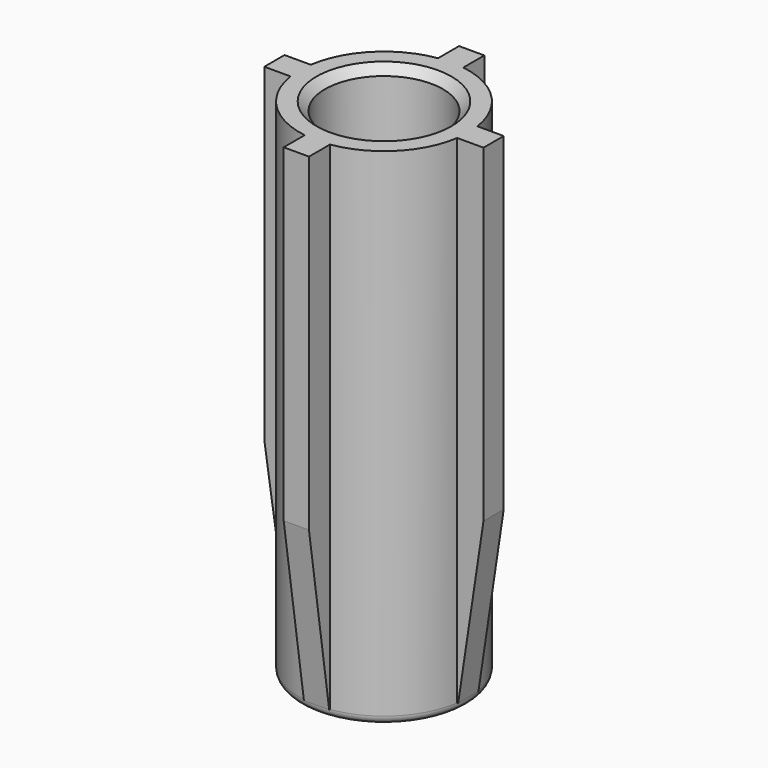
from build123d import *

# Parameters (mm, degrees)
F1_R        = 5
F1_R_2      = 3.5
F2_DEPTH    = 30
F4_W        = 1.5
F4_H        = 2.639524132
F5_DEPTH    = 29.5
F6_COUNT    = 4
F8_R        = 3.5
F8_R_2      = 1.75
F9_DEPTH    = 1.5
F10_SIZE2   = 1.49999
F10_SIZE    = 9.99999
F10_2_SIZE2 = 1.49999
F10_2_SIZE  = 9.99999
F10_3_SIZE2 = 1.49999
F10_3_SIZE  = 9.99999
F10_4_SIZE2 = 1.49999
F10_4_SIZE  = 9.99999
F11_SIZE    = 0.5
F12_R       = 0.49999


# Not quite as in the source:
# - a fillet or chamfer is up to 0.001 mm smaller than in the source, because OpenCascade refuses the exact size


with BuildPart() as f2:
    # F1 (on offset) → F2 (new body)
    with BuildSketch(Plane.XY):
        with Locations((-25, 25)):
            Circle(F1_R)
        with Locations((-25, 25)):
            Circle(F1_R_2, mode=Mode.SUBTRACT)
    extrude(amount=-F2_DEPTH)

    # F4 (on offset) → F5 (join)
    with BuildSketch(Plane.XY):
        with Locations((-25, 30.180237934)):
            Rectangle(F4_W, F4_H)
    extrude(amount=-F5_DEPTH)

    # F6: F2 ×4 about axis
    f6_axis = Axis((-25, 25, 0), (0, 0, 1))


with BuildPart() as f2_1:
    add(f2.part)
    for i in range(1, F6_COUNT):
        add(f2.part.rotate(f6_axis, i * 360 / F6_COUNT))

    # F8 (on offset) → F9 (join)
    with BuildSketch(Plane.XY.offset(-30)):
        with Locations((-25, 25)):
            Circle(F8_R)
        with Locations((-25, 25)):
            Circle(F8_R_2, mode=Mode.SUBTRACT)
    extrude(amount=F9_DEPTH)

    # F10 (size 10 and 1.5 in the source; OpenCascade refuses exactly that, so slightly less here)
    f10_edges = [f2_1.edges().sort_by_distance(p)[0] for p in [
        (-25, 18.5, -29.5),
    ]]
    f10_side = f2_1.faces().sort_by_distance((-25, 18.5, -14.75))[0]
    chamfer(f10_edges, length=F10_SIZE, length2=F10_SIZE2, reference=f10_side)

    # F10#2 (size 10 and 1.5 in the source; OpenCascade refuses exactly that, so slightly less here)
    f10_2_edges = [f2_1.edges().sort_by_distance(p)[0] for p in [
        (-18.5, 25, -29.5),
    ]]
    f10_2_side = f2_1.faces().sort_by_distance((-18.5, 25, -14.75))[0]
    chamfer(f10_2_edges, length=F10_2_SIZE, length2=F10_2_SIZE2, reference=f10_2_side)

    # F10#3 (size 10 and 1.5 in the source; OpenCascade refuses exactly that, so slightly less here)
    f10_3_edges = [f2_1.edges().sort_by_distance(p)[0] for p in [
        (-25, 31.5, -29.5),
    ]]
    f10_3_side = f2_1.faces().sort_by_distance((-25, 31.5, -14.75))[0]
    chamfer(f10_3_edges, length=F10_3_SIZE, length2=F10_3_SIZE2, reference=f10_3_side)

    # F10#4 (size 10 and 1.5 in the source; OpenCascade refuses exactly that, so slightly less here)
    f10_4_edges = [f2_1.edges().sort_by_distance(p)[0] for p in [
        (-31.5, 25, -29.5),
    ]]
    f10_4_side = f2_1.faces().sort_by_distance((-31.5, 25, -14.75))[0]
    chamfer(f10_4_edges, length=F10_4_SIZE, length2=F10_4_SIZE2, reference=f10_4_side)

    # F11
    f11_edges = [f2_1.edges().sort_by_distance(p)[0] for p in [
        (-28.5, 25, 0),
        (-26.75, 25, -28.5),
    ]]
    chamfer(f11_edges, length=F11_SIZE)

    # F12 (radius 0.5 in the source; OpenCascade refuses exactly that, so slightly less here)
    f12_edges = [f2_1.edges().sort_by_distance(p)[0] for p in [
        (-30, 25, -30),
    ]]
    fillet(f12_edges, radius=F12_R)


solid = f2_1.part
